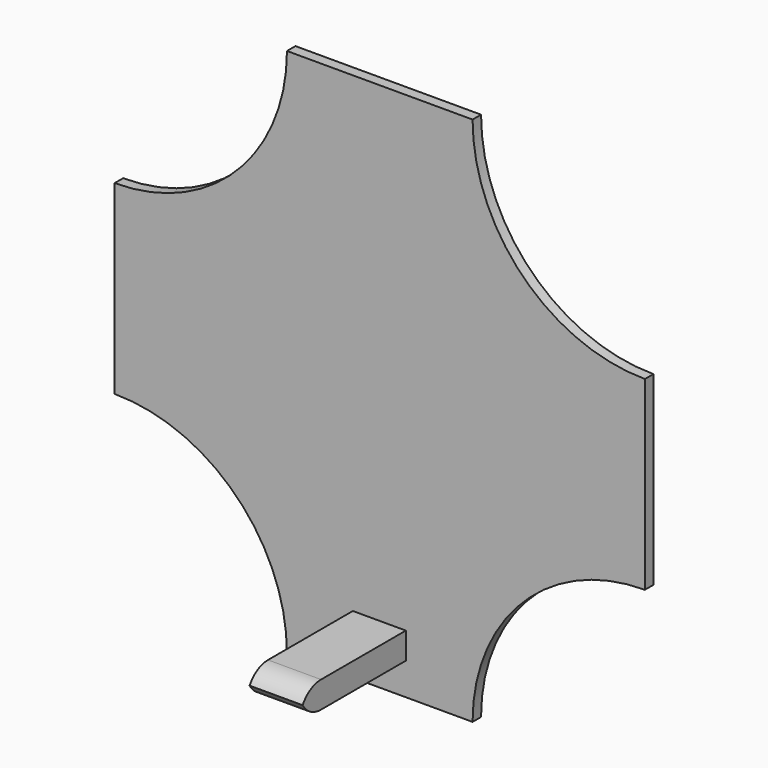
from build123d import *

# Parameters (mm, degrees)
F0_W        = 100
F0_H        = 100
F1_DEPTH    = 2
F3_DEPTH    = 25
F5_DEPTH    = 25
F6_W        = 10
F6_H        = 5
F7_DEPTH    = 25
F8_T1_DEPTH = 35


# Not quite as in the source:
# - a fillet or chamfer that OpenCascade refuses, or shapes differently, is made with other operations: its cross-section is extruded or revolved along the edge and cut away or added


with BuildPart() as f1:
    # F0 (on Front) → F1 (new body)
    with BuildSketch(Plane.XZ):
        with Locations((-22.4419460681, 3.9658267051)):
            Rectangle(F0_W, F0_H)
    extrude(amount=F1_DEPTH)

    # F2 (on face) → F3 (cut)
    with BuildSketch(Plane.XZ.offset(2)):
        with BuildLine():
            ThreePointArc((-72.4419460681, -13.5341732949), (-95.4229164567, -69.0151436835), (-39.9419460681, -46.0341732949))
            Line((-39.9419460681, -46.0341732949), (-72.4419460681, -46.0341732949))
            Line((-72.4419460681, -46.0341732949), (-72.4419460681, -13.5341732949))
        make_face()
        with BuildLine():
            Line((-72.4419460681, 53.9658267051), (-39.9419460681, 53.9658267051))
            ThreePointArc((-39.9419460681, 53.9658267051), (-95.4229164567, 76.9467970937), (-72.4419460681, 21.4658267051))
            Line((-72.4419460681, 21.4658267051), (-72.4419460681, 53.9658267051))
        make_face()
        with BuildLine():
            ThreePointArc((-72.4419460681, 21.4658267051), (-49.4609756796, 30.9848563165), (-39.9419460681, 53.9658267051))
            Line((-39.9419460681, 53.9658267051), (-72.4419460681, 53.9658267051))
            Line((-72.4419460681, 53.9658267051), (-72.4419460681, 21.4658267051))
        make_face()
        with BuildLine():
            Line((27.5580539319, 53.9658267051), (27.5580539319, 21.4658267051))
            ThreePointArc((27.5580539319, 21.4658267051), (50.5390243204, 30.9848563165), (60.0580539319, 53.9658267051))
            ThreePointArc((60.0580539319, 53.9658267051), (27.5580539319, 86.4658267051), (-4.9419460681, 53.9658267051))
            Line((-4.9419460681, 53.9658267051), (27.5580539319, 53.9658267051))
        make_face()
        with BuildLine():
            ThreePointArc((-4.9419460681, 53.9658267051), (4.5770835433, 30.9848563165), (27.5580539319, 21.4658267051))
            Line((27.5580539319, 21.4658267051), (27.5580539319, 53.9658267051))
            Line((27.5580539319, 53.9658267051), (-4.9419460681, 53.9658267051))
        make_face()
        with BuildLine():
            ThreePointArc((-4.9419460681, -46.0341732949), (27.5580539319, -78.5341732949), (60.0580539319, -46.0341732949))
            ThreePointArc((60.0580539319, -46.0341732949), (50.5390243204, -23.0532029063), (27.5580539319, -13.5341732949))
            Line((27.5580539319, -13.5341732949), (27.5580539319, -46.0341732949))
            Line((27.5580539319, -46.0341732949), (-4.9419460681, -46.0341732949))
        make_face()
        with BuildLine():
            Line((27.5580539319, -46.0341732949), (27.5580539319, -13.5341732949))
            ThreePointArc((27.5580539319, -13.5341732949), (4.5770835433, -23.0532029063), (-4.9419460681, -46.0341732949))
            Line((-4.9419460681, -46.0341732949), (27.5580539319, -46.0341732949))
        make_face()
    extrude(amount=-F3_DEPTH, mode=Mode.SUBTRACT)

    # F4 (on face) → F5 (cut)
    with BuildSketch(Plane.XZ.offset(2)):
        with BuildLine():
            ThreePointArc((-72.4419460681, -13.5341732949), (-95.4229164567, -69.0151436835), (-39.9419460681, -46.0341732949))
            Line((-39.9419460681, -46.0341732949), (-72.4419460681, -46.0341732949))
            Line((-72.4419460681, -46.0341732949), (-72.4419460681, -13.5341732949))
        make_face()
        with BuildLine():
            Line((-72.4419460681, -46.0341732949), (-39.9419460681, -46.0341732949))
            ThreePointArc((-39.9419460681, -46.0341732949), (-49.4609756796, -23.0532029063), (-72.4419460681, -13.5341732949))
            Line((-72.4419460681, -13.5341732949), (-72.4419460681, -46.0341732949))
        make_face()
    extrude(amount=-F5_DEPTH, mode=Mode.SUBTRACT)

    # F6 (on face) → F7 (join)
    with BuildSketch(Plane.XZ.offset(2)):
        with Locations((-22.5202348083, -37.4598563993)):
            Rectangle(F6_W, F6_H)
    extrude(amount=F7_DEPTH)

    # F8: fillet of radius 5 on 2 edges, made by hand

    # F8_s2 → F8_t1 (cut)
    with BuildSketch(Plane.YZ.offset(-40.0202348083)):
        with BuildLine():
            ThreePointArc((-22, -34.9598563993), (-25.5355339059, -36.4243224934), (-27, -39.9598563993))
            Line((-27, -39.9598563993), (-27, -34.9598563993))
            Line((-27, -34.9598563993), (-22, -34.9598563993))
        make_face()
        with BuildLine():
            ThreePointArc((-22, -39.9598563993), (-25.5355339059, -38.4953903053), (-27, -34.9598563993))
            Line((-27, -34.9598563993), (-27, -39.9598563993))
            Line((-27, -39.9598563993), (-22, -39.9598563993))
        make_face()
    extrude(amount=F8_T1_DEPTH, mode=Mode.SUBTRACT)


solid = f1.part
